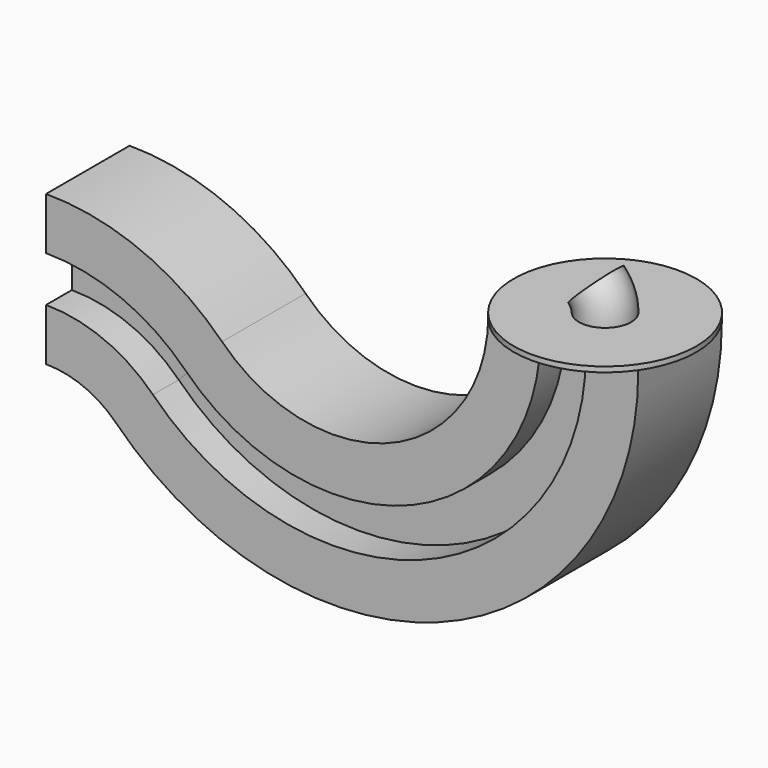
from build123d import *

# Parameters (mm, degrees)
F0_R     = 5
F1_ANGLE = 45
F2_R     = 17.5
F2_R_2   = 5
F3_DEPTH = 1
F5_ANGLE = 135
F7_ANGLE = 45


with BuildPart() as f1:
    # F0 (on Top) → F1 (revolve)
    with BuildSketch(Plane.XY):
        with Locations((17.2625295818, 39.9485491216)):
            Circle(F0_R)
    revolve(axis=Axis((11.3439466804, 38.7977138162, 0), (0, -1, 0)), revolution_arc=F1_ANGLE)

    # F2 (on face) → F3 (join)
    with BuildSketch(Plane(origin=(0, 0, 0), x_dir=(1, 0, 0), z_dir=(0, 0, -1))):
        with Locations((17.2625295818, -39.9485491216)):
            Circle(F2_R)
        with Locations((17.2625295818, -39.9485491216)):
            Circle(F2_R_2, mode=Mode.SUBTRACT)
        with Locations((17.2625295818, -39.9485491216)):
            Circle(F2_R_2)
    extrude(amount=F3_DEPTH)

    # F4 (on face) → F5 (revolve)
    with BuildSketch(Plane(origin=(0, 0, -1), x_dir=(1, 0, 0), z_dir=(0, 0, -1))):
        Polygon((12.9011229654, -29.9485491216), (2.9011229654, -29.9485491216), (2.9011229654, -49.9485491216), (12.9011229654, -49.9485491216), (12.9011229654, -44.1824280606), (21.6239361981, -44.1824280606), (21.6239361981, -49.9485491216), (31.6239361981, -49.9485491216), (31.6239361981, -29.9485491216), (21.6239361981, -29.9485491216), (21.6239361981, -36.1191299331), (12.9011229654, -36.1218505295), align=None)
    revolve(axis=Axis((-26.9732894376, 40.484293364, -1), (0, 1, 0)), revolution_arc=F5_ANGLE)

    # F6 (on face) → F7 (revolve)
    with BuildSketch(Plane(origin=(-12.9866447188, 0, 12.9866447188), x_dir=(0, -1, 0), z_dir=(-0.7071067812, 0, 0.7071067812))):
        Polygon((-36.1218505295, -59.6545150564), (-29.9485491216, -59.6545150564), (-29.9485491216, -49.6545150564), (-49.9485491216, -49.6545150564), (-49.9485491216, -59.6545150564), (-44.1824280606, -59.6545150564), (-44.1824280606, -68.3773282891), (-49.9485491216, -68.3773282891), (-49.9485491216, -78.3773282891), (-29.9485491216, -78.3773282891), (-29.9485491216, -68.3773282891), (-36.1191299331, -68.3773282891), align=None)
    revolve(axis=Axis((-81.8073011532, 42.3686988652, -55.8340117156), (0, -1, 0)), revolution_arc=F7_ANGLE)


solid = f1.part
